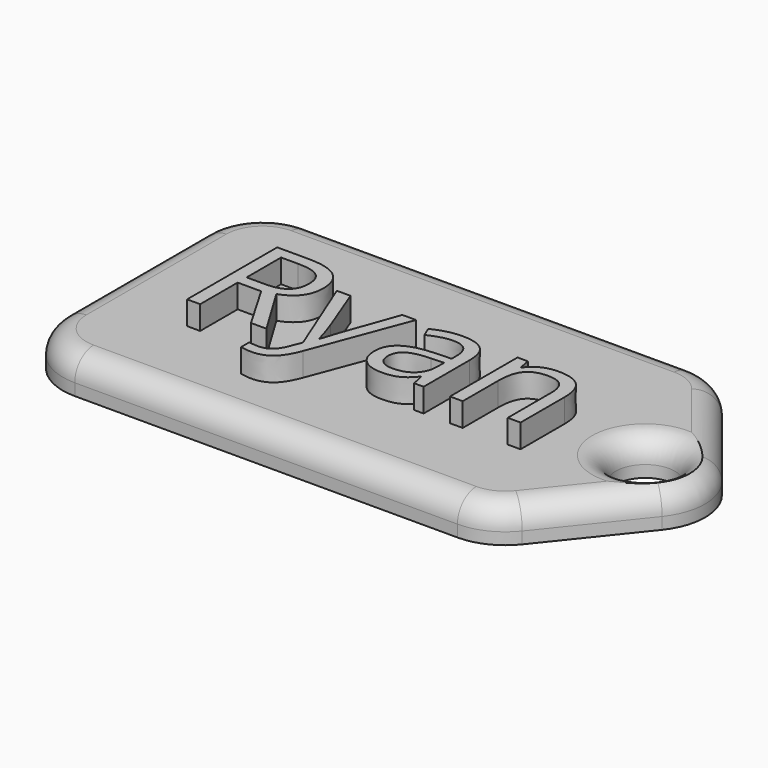
from build123d import *

# Parameters (mm, degrees)
F1_DEPTH     = 3
F2_R         = 5.08
F4_D         = 5
F5_R         = 5.08
F6_T1_DEPTH  = 32.4784257748
F6_T3_DEPTH  = 14.84
F6_T5_DEPTH  = 9.5022363684
F6_T7_DEPTH  = 9.5022363684
F6_T10_ANGLE = 90
F6_T12_ANGLE = 51.3401917459
F6_T14_ANGLE = 90
F6_T16_ANGLE = 77.3196165082
F6_T18_ANGLE = 51.3401917459
F7_TEXT_SIZE = 13.3904448105
F8_DEPTH     = 2


# Not quite as in the source:
# - a fillet or chamfer that OpenCascade refuses, or shapes differently, is made with other operations: its cross-section is extruded or revolved along the edge and cut away or added
# - Text() gives the source's letters only with a copy of the font that has no kerning and outlines rounded to 1/6400 em; it was checked with that copy


with BuildPart() as f1:
    # F0 (on Top) → F1 (new body)
    with BuildSketch(Plane.XY):
        Polygon((-20, -12.5), (20, -12.5), (30, 0), (20, 12.5), (-20, 12.5), align=None)
    extrude(amount=F1_DEPTH)

    # F2
    f2_edges = [f1.edges().sort_by_distance(p)[0] for p in [
        (20, -12.5, 1.5),
        (30, 0, 1.5),
        (20, 12.5, 1.5),
    ]]
    fillet(f2_edges, radius=F2_R)

    # F4 (through all)
    with Locations(Plane.XY.offset(3)):
        with Locations((23.4944257748, 0)):
            Hole(F4_D / 2)

    # F5
    f5_edges = [f1.edges().sort_by_distance(p)[0] for p in [
        (-20, 12.5, 1.5),
        (-20, -12.5, 1.5),
    ]]
    fillet(f5_edges, radius=F5_R)

    # F6: fillet of radius 2 on 11 edges, made by hand

    # F6_s2 → F6_t1 (cut)
    with BuildSketch(Plane.YZ.offset(-14.92)):
        with BuildLine():
            ThreePointArc((-12.5, 1), (-11.9142135624, 2.4142135624), (-10.5, 3))
            Line((-10.5, 3), (-12.5, 3))
            Line((-12.5, 3), (-12.5, 1))
        make_face()
        with BuildLine():
            ThreePointArc((10.5, 3), (11.9142135624, 2.4142135624), (12.5, 1))
            Line((12.5, 1), (12.5, 3))
            Line((12.5, 3), (10.5, 3))
        make_face()
    extrude(amount=F6_T1_DEPTH, mode=Mode.SUBTRACT)

    # F6_s4 → F6_t3 (cut)
    with BuildSketch(Plane.XZ.offset(-7.42)):
        with BuildLine():
            ThreePointArc((-18, 3), (-19.4142135624, 2.4142135624), (-20, 1))
            Line((-20, 1), (-20, 3))
            Line((-20, 3), (-18, 3))
        make_face()
    extrude(amount=F6_T3_DEPTH, mode=Mode.SUBTRACT)

    # F6_s6 → F6_t5 (cut)
    with BuildSketch(Plane(origin=(3.2325563999, 4.0406954999, 0), x_dir=(0, 0, 1), z_dir=(0.6246950476, 0.7808688094, 0))):
        with BuildLine():
            ThreePointArc((3, 21.4260642833), (2.4142135624, 22.8402778457), (1, 23.4260642833))
            Line((1, 23.4260642833), (3, 23.4260642833))
            Line((3, 23.4260642833), (3, 21.4260642833))
        make_face()
    extrude(amount=F6_T5_DEPTH, mode=Mode.SUBTRACT)

    # F6_s8 → F6_t7 (cut)
    with BuildSketch(Plane(origin=(9.1685563999, -11.4606954999, 0), x_dir=(0, 0, 1), z_dir=(-0.6246950476, 0.7808688094, 0))):
        with BuildLine():
            ThreePointArc((3, 21.4260642833), (2.4142135624, 22.8402778457), (1, 23.4260642833))
            Line((1, 23.4260642833), (3, 23.4260642833))
            Line((3, 23.4260642833), (3, 21.4260642833))
        make_face()
    extrude(amount=F6_T7_DEPTH, mode=Mode.SUBTRACT)

    # F6_s9 → F6_t10 (revolve, cut)
    with BuildSketch(Plane.YZ.offset(-14.92)):
        with BuildLine():
            ThreePointArc((-12.5, 1), (-11.9142135624, 2.4142135624), (-10.5, 3))
            Line((-10.5, 3), (-12.5, 3))
            Line((-12.5, 3), (-12.5, 1))
        make_face()
    revolve(axis=Axis((-14.92, -7.42, 3), (0, 0, -1)), revolution_arc=F6_T10_ANGLE, mode=Mode.SUBTRACT)

    # F6_s11 → F6_t12 (revolve, cut)
    with BuildSketch(Plane.YZ.offset(17.5584257748)):
        with BuildLine():
            ThreePointArc((-12.5, 1), (-11.9142135624, 2.4142135624), (-10.5, 3))
            Line((-10.5, 3), (-12.5, 3))
            Line((-12.5, 3), (-12.5, 1))
        make_face()
    revolve(axis=Axis((17.5584257748, -7.42, 3), (0, 0, 1)), revolution_arc=F6_T12_ANGLE, mode=Mode.SUBTRACT)

    # F6_s13 → F6_t14 (revolve, cut)
    with BuildSketch(Plane.XZ.offset(-7.42)):
        with BuildLine():
            ThreePointArc((-18, 3), (-19.4142135624, 2.4142135624), (-20, 1))
            Line((-20, 1), (-20, 3))
            Line((-20, 3), (-18, 3))
        make_face()
    revolve(axis=Axis((-14.92, 7.42, 3), (0, 0, -1)), revolution_arc=F6_T14_ANGLE, mode=Mode.SUBTRACT)

    # F6_s15 → F6_t16 (revolve, cut)
    with BuildSketch(Plane(origin=(9.1685563999, 11.4606954999, 0), x_dir=(0, 0, 1), z_dir=(-0.6246950476, -0.7808688094, 0))):
        with BuildLine():
            ThreePointArc((3, -21.4260642833), (2.4142135624, -22.8402778457), (1, -23.4260642833))
            Line((1, -23.4260642833), (3, -23.4260642833))
            Line((3, -23.4260642833), (3, -21.4260642833))
        make_face()
    revolve(axis=Axis((23.4944257748, 0, 3), (0, 0, 1)), revolution_arc=F6_T16_ANGLE, mode=Mode.SUBTRACT)

    # F6_s17 → F6_t18 (revolve, cut)
    with BuildSketch(Plane(origin=(3.2325563999, -4.0406954999, 0), x_dir=(0, 0, 1), z_dir=(0.6246950476, -0.7808688094, 0))):
        with BuildLine():
            ThreePointArc((3, -21.4260642833), (2.4142135624, -22.8402778457), (1, -23.4260642833))
            Line((1, -23.4260642833), (3, -23.4260642833))
            Line((3, -23.4260642833), (3, -21.4260642833))
        make_face()
    revolve(axis=Axis((17.5584257748, 7.42, 3), (0, 0, 1)), revolution_arc=F6_T18_ANGLE, mode=Mode.SUBTRACT)

    # F6_s19 → F6_t20 (revolve, cut)
    with BuildSketch(Plane.XZ):
        with BuildLine():
            ThreePointArc((27.9944257748, 3), (26.5802122124, 2.4142135624), (25.9944257748, 1))
            Line((25.9944257748, 1), (25.9944257748, 3))
            Line((25.9944257748, 3), (27.9944257748, 3))
        make_face()
    revolve(axis=Axis((23.4944257748, 0, 3), (0, 0, 1)), mode=Mode.SUBTRACT)

    # F7 (on face) → F8 (join)
    with BuildSketch(Plane.XY.offset(3)):
        with Locations((-13.096370489, -4.5062846778)):
            Text('Ryan', F7_TEXT_SIZE, font='Open Sans', text_align=(TextAlign.LEFT, TextAlign.BOTTOM))
    extrude(amount=F8_DEPTH)


solid = f1.part
